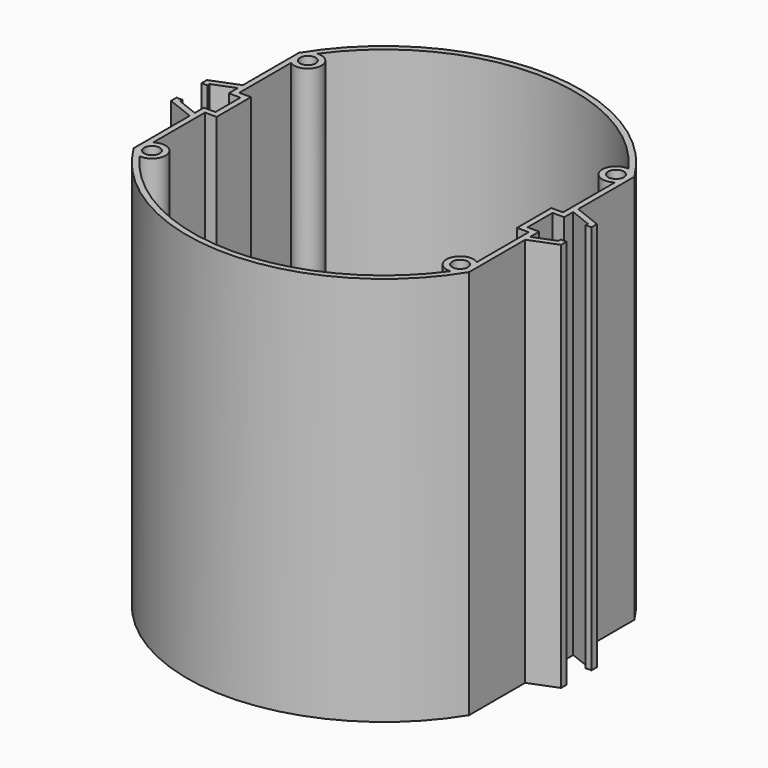
from build123d import *

# Parameters (mm, degrees)
F0_R          = 2
F1_DEPTH      = 100
F1_DEPTH_BACK = 1.5
F2_T          = 1.5
F2_T3_DEPTH   = 104.5
F0_W          = 7
F0_H          = 1.75
F0_H_2        = 8
F0_W_2        = 3
F3_DEPTH      = 100
F3_DEPTH_BACK = 1.5
F4_T          = 1.5
F4_T3_DEPTH   = 104.5
F4_T5_DEPTH   = 103
F4_T7_DEPTH   = 19.6088440305
F4_T9_DEPTH   = 6
F4_T11_DEPTH  = 14
F4_T13_DEPTH  = 19.6088440305
F4_T15_DEPTH  = 6
F4_T18_ANGLE  = 221.2149297422
F4_T20_ANGLE  = 108.9853327241
F4_T22_ANGLE  = 221.2149297422
F4_T24_ANGLE  = 221.2149297422
F4_T26_ANGLE  = 108.9853327241
F4_T28_ANGLE  = 221.2149297422
F0_W_3        = 2
F5_DEPTH      = 1.5
F6_DEPTH      = 100
F6_DEPTH_BACK = 1.5


# Not quite as in the source:
# - a shell that OpenCascade refuses in one call is made with other operations: the cavity is built on its own and cut out


with BuildPart() as f1:
    # F0 (on Top) → F1 (new body, two sides)
    with BuildSketch(Plane.XY) as f1_sk:
        with BuildLine():
            Line((43, 8.5), (43, 26.4811253537))
            ThreePointArc((43, 26.4811253537), (0, 50.5), (-43, 26.4811253537))
            Line((-43, 26.4811253537), (-43, 8.5))
            Line((-43, 8.5), (-43, 5.75))
            Line((-43, 5.75), (-43, 4))
            Line((-43, 4), (-40, 4))
            Line((-40, 4), (-40, -4))
            Line((-40, -4), (-43, -4))
            Line((-43, -4), (-43, -5.75))
            Line((-43, -5.75), (-43, -8.5))
            Line((-43, -8.5), (-43, -26.4811253537))
            ThreePointArc((-43, -26.4811253537), (0, -50.5), (43, -26.4811253537))
            Line((43, -26.4811253537), (43, -8.5))
            Line((43, -8.5), (43, -5.75))
            Line((43, -5.75), (43, -4))
            Line((43, -4), (40, -4))
            Line((40, -4), (40, 4))
            Line((40, 4), (43, 4))
            Line((43, 4), (43, 5.75))
            Line((43, 5.75), (43, 8.5))
        make_face()
        with Locations((-39.5, -24.9811253537)):
            Circle(F0_R, mode=Mode.SUBTRACT)
        with Locations((39.5, -24.9811253537)):
            Circle(F0_R, mode=Mode.SUBTRACT)
        with Locations((-39.5, 24.9811253537)):
            Circle(F0_R, mode=Mode.SUBTRACT)
        with Locations((39.5, 24.9811253537)):
            Circle(F0_R, mode=Mode.SUBTRACT)
    extrude(amount=F1_DEPTH)
    extrude(f1_sk.sketch, amount=-F1_DEPTH_BACK)

    # F2: shell of thickness 1.5, made by hand


with BuildPart() as f2_core1:
    # F2_t2: copy of F1
    add(f1.part)

    # the walls: a layer under each face that stays
    f2_faces = [f2_core1.faces().sort_by_distance(p)[0] for p in [
        (43, -15.2405626769, 49.25),
        (0, 0, -1.5),
        (37.5, 24.9811253537, 49.25),
        (-41.5, 24.9811253537, 49.25),
        (37.5, -24.9811253537, 49.25),
        (-41.5, -24.9811253537, 49.25),
        (-43, -15.2405626769, 49.25),
        (-41.5, -4, 49.25),
        (-40, 0, 49.25),
        (-41.5, 4, 49.25),
        (-43, 15.2405626769, 49.25),
        (0, 50.5, 49.25),
        (43, 15.2405626769, 49.25),
        (41.5, 4, 49.25),
        (40, 0, 49.25),
        (41.5, -4, 49.25),
        (0, -50.5, 49.25),
    ]]
    thicken(f2_faces, amount=-F2_T, mode=Mode.SUBTRACT)

    # F2_s4 → F2_t3 (cut)
    with BuildSketch(Plane.XY.offset(-3)):
        Polygon((-40.015, -3.985), (-40, -5.5), (-38.5, -5.5), (-38.5, -4), align=None)
        Polygon((-40.015, 3.985), (-38.5, 4), (-38.5, 5.5), (-40, 5.5), align=None)
        Polygon((40.015, 3.985), (40, 5.5), (38.5, 5.5), (38.5, 4), align=None)
        Polygon((40.015, -3.985), (38.5, -4), (38.5, -5.5), (40, -5.5), align=None)
    extrude(amount=F2_T3_DEPTH, mode=Mode.SUBTRACT)


with BuildPart() as f1_1:
    add(f1.part)

    # what is left inside the walls is the cavity
    f2_cavity = [f2_core1.part.solids().sort_by_distance(p)[0] for p in [
        (0, -48.985, 66.666667),
    ]]
    add(f2_cavity, mode=Mode.SUBTRACT)

    # F0 (on Top) → F3 (join, two sides)
    with BuildSketch(Plane.XY) as f3_sk:
        Polygon((-43, 5.75), (-43, 8.5), (-50, 5.75), align=None)
        with Locations((-46.5, 4.875)):
            Rectangle(F0_W, F0_H)
        with Locations((-46.5, 0)):
            Rectangle(F0_W, F0_H_2)
        with Locations((-46.5, -4.875)):
            Rectangle(F0_W, F0_H)
        Polygon((-43, -8.5), (-43, -5.75), (-50, -5.75), align=None)
        with Locations((-41.5, 0)):
            Rectangle(F0_W_2, F0_H_2)
        Polygon((50, -5.75), (43, -5.75), (43, -8.5), align=None)
        with Locations((46.5, -4.875)):
            Rectangle(F0_W, F0_H)
        with Locations((46.5, 0)):
            Rectangle(F0_W, F0_H_2)
        with Locations((41.5, 0)):
            Rectangle(F0_W_2, F0_H_2)
        Polygon((50, 5.75), (43, 8.5), (43, 5.75), align=None)
        with Locations((46.5, 4.875)):
            Rectangle(F0_W, F0_H)
    extrude(amount=F3_DEPTH)
    extrude(f3_sk.sketch, amount=-F3_DEPTH_BACK)

    # F4: shell of thickness 1.5, made by hand


with BuildPart() as f4_core1:
    # F4_t2: copy of F1
    add(f1_1.part)

    # the walls: a layer under each face that stays
    f4_faces = [f4_core1.faces().sort_by_distance(p)[0] for p in [
        (43, -17.4905626769, 49.25),
        (0, -50.5, 49.25),
        (0, 0, -1.5),
        (46.5, -7.125, 49.25),
        (-43, -17.4905626769, 49.25),
        (43, 17.4905626769, 49.25),
        (0, 50.5, 49.25),
        (-43, 17.4905626769, 49.25),
        (-41.5, -24.9811253537, 49.25),
        (37.5, -24.9811253537, 49.25),
        (-41.5, 24.9811253537, 49.25),
        (37.5, 24.9811253537, 49.25),
        (50, 0, 49.25),
        (41.5, -13.8044220152, 50),
        (40, -5.5, 50),
        (38.5, 0, 50),
        (40, 5.5, 50),
        (41.5, 13.8044220152, 50),
        (36.1075781641, 24.1200364574, 50),
        (0, 49, 50),
        (-36.1075781641, 24.1200364574, 50),
        (-41.5, 13.8044220152, 50),
        (-40, 5.5, 50),
        (-38.5, 0, 50),
        (-40, -5.5, 50),
        (-41.5, -13.8044220152, 50),
        (-36.1075781641, -24.1200364574, 50),
        (0, -49, 50),
        (36.1075781641, -24.1200364574, 50),
        (-46.5, -7.125, 49.25),
        (46.5, 7.125, 49.25),
        (-46.5, 7.125, 49.25),
        (-50, 0, 49.25),
        (0, 0, 0),
    ]]
    thicken(f4_faces, amount=-F4_T, mode=Mode.SUBTRACT)

    # F4_s4 → F4_t3 (cut)
    with BuildSketch(Plane.XY.offset(-3)):
        Polygon((43.0204847856, -8.5139612724), (41.5, -8.5), (41.5, -7.4776847547), (42.4515214414, -7.1038727598), align=None)
        Polygon((-43.0204847856, -8.5139612724), (-41.5, -8.5), (-41.5, -7.4776847547), (-42.4515214414, -7.1038727598), align=None)
        Polygon((43.0204847856, 8.5139612724), (41.5, 8.5), (41.5, 7.4776847547), (42.4515214414, 7.1038727598), align=None)
        Polygon((-43.0204847856, 8.5139612724), (-41.5, 8.5), (-41.5, 7.4776847547), (-42.4515214414, 7.1038727598), align=None)
    extrude(amount=F4_T3_DEPTH, mode=Mode.SUBTRACT)

    # F4_s6 → F4_t5 (cut)
    with BuildSketch(Plane.XY.offset(-1.5)):
        Polygon((41.4935714286, -22.0965342534), (43, -22.1088440305), (43, -24.9811253537), (40.6428571429, -23.3398217404), align=None)
        Polygon((41.485, -5.515), (43, -5.5), (43, -4), (41.5, -4), align=None)
        Polygon((41.485, 5.515), (41.5, 4), (43, 4), (43, 5.5), align=None)
        Polygon((41.4935714286, 22.0965342534), (43, 22.1088440305), (43, 24.9811253537), (40.6428571429, 23.3398217404), align=None)
        Polygon((39.8774703303, 28.4657460045), (39.7217245792, 26.9687969088), (43.0599998648, 26.5964126076), (41.1090797896, 29.330761307), align=None)
        Polygon((-39.8774703303, 28.4657460045), (-41.1090797896, 29.330761307), (-43.0599998648, 26.5964126076), (-39.7217245792, 26.9687969088), align=None)
        Polygon((-41.4935714286, 22.0965342534), (-40.6428571429, 23.3398217404), (-43, 24.9811253537), (-43, 22.1088440305), align=None)
        Polygon((-41.485, 5.515), (-43, 5.5), (-43, 4), (-41.5, 4), align=None)
        Polygon((-41.485, -5.515), (-41.5, -4), (-43, -4), (-43, -5.5), align=None)
        Polygon((-41.4935714286, -22.0965342534), (-43, -22.1088440305), (-43, -24.9811253537), (-40.6428571429, -23.3398217404), align=None)
        Polygon((-39.8774703303, -28.4657460045), (-39.7217245792, -26.9687969088), (-43.0599998648, -26.5964126076), (-41.1090797896, -29.330761307), align=None)
        Polygon((39.8774703303, -28.4657460045), (41.1090797896, -29.330761307), (43.0599998648, -26.5964126076), (39.7217245792, -26.9687969088), align=None)
    extrude(amount=F4_T5_DEPTH, mode=Mode.SUBTRACT)

    # F4_s8 → F4_t7 (cut)
    with BuildSketch(Plane.XZ.offset(4)):
        Polygon((41.485, 0.015), (43, 0), (43, -1.5), (41.5, -1.5), align=None)
        Polygon((-41.485, 0.015), (-43, 0), (-43, -1.5), (-41.5, -1.5), align=None)
    extrude(amount=F4_T7_DEPTH, mode=Mode.SUBTRACT)

    # F4_s10 → F4_t9 (cut)
    with BuildSketch(Plane.YZ.offset(37)):
        Polygon((-5.515, 0.015), (-4, 0), (-4, -1.5), (-5.5, -1.5), align=None)
        Polygon((5.515, 0.015), (4, 0), (4, -1.5), (5.5, -1.5), align=None)
    extrude(amount=F4_T9_DEPTH, mode=Mode.SUBTRACT)

    # F4_s12 → F4_t11 (cut)
    with BuildSketch(Plane.XZ.offset(-7)):
        Polygon((38.485, 0.015), (40, 0), (40, -1.5), (38.5, -1.5), align=None)
        Polygon((-38.485, 0.015), (-40, 0), (-40, -1.5), (-38.5, -1.5), align=None)
    extrude(amount=F4_T11_DEPTH, mode=Mode.SUBTRACT)

    # F4_s14 → F4_t13 (cut)
    with BuildSketch(Plane.XZ.offset(-23.6088440305)):
        Polygon((41.485, 0.015), (43, 0), (43, -1.5), (41.5, -1.5), align=None)
        Polygon((-41.485, 0.015), (-43, 0), (-43, -1.5), (-41.5, -1.5), align=None)
    extrude(amount=F4_T13_DEPTH, mode=Mode.SUBTRACT)

    # F4_s16 → F4_t15 (cut)
    with BuildSketch(Plane.YZ.offset(-43)):
        Polygon((5.515, 0.015), (4, 0), (4, -1.5), (5.5, -1.5), align=None)
        Polygon((-5.515, 0.015), (-4, 0), (-4, -1.5), (-5.5, -1.5), align=None)
    extrude(amount=F4_T15_DEPTH, mode=Mode.SUBTRACT)

    # F4_s17 → F4_t18 (revolve, cut)
    with BuildSketch(Plane(origin=(38.3167869041, 26.6803857921, 0), x_dir=(0, 0, 1), z_dir=(0.8206518066, 0.5714285714, 0))):
        Polygon((0.015, 5.5856229178), (0, 4.0706229178), (-1.5, 4.0706229178), (-1.5, 5.5706229178), align=None)
    revolve(axis=Axis((39.5, 24.9811253537, 0), (0, 0, -1)), revolution_arc=F4_T18_ANGLE, mode=Mode.SUBTRACT)

    # F4_s19 → F4_t20 (revolve, cut)
    with BuildSketch(Plane(origin=(0, 0, 0), x_dir=(0, 0, 1), z_dir=(-0.5808071546, -0.814041184, 0))):
        Polygon((0.015, 48.985), (0, 50.5), (-1.5, 50.5), (-1.5, 49), align=None)
    revolve(axis=Axis((0, 0, 0), (0, 0, -1)), revolution_arc=F4_T20_ANGLE, mode=Mode.SUBTRACT)

    # F4_s21 → F4_t22 (revolve, cut)
    with BuildSketch(Plane(origin=(-38.3167869041, 26.6803857921, 0), x_dir=(0, 0, 1), z_dir=(-0.8206518066, 0.5714285714, 0))):
        Polygon((0.015, -5.5856229178), (0, -4.0706229178), (-1.5, -4.0706229178), (-1.5, -5.5706229178), align=None)
    revolve(axis=Axis((-39.5, 24.9811253537, 0), (0, 0, 1)), revolution_arc=F4_T22_ANGLE, mode=Mode.SUBTRACT)

    # F4_s23 → F4_t24 (revolve, cut)
    with BuildSketch(Plane(origin=(-36.2621341759, 4.0450377338, 0), x_dir=(0, 0, 1), z_dir=(-0.9938357776, 0.1108622896, 0))):
        Polygon((0.015, -32.7211965802), (0, -31.2061965802), (-1.5, -31.2061965802), (-1.5, -32.7061965802), align=None)
    revolve(axis=Axis((-39.5, -24.9811253537, 0), (0, 0, 1)), revolution_arc=F4_T24_ANGLE, mode=Mode.SUBTRACT)

    # F4_s25 → F4_t26 (revolve, cut)
    with BuildSketch(Plane(origin=(0, 0, 0), x_dir=(0, 0, 1), z_dir=(0.5808071546, 0.814041184, 0))):
        Polygon((0.015, 48.985), (0, 50.5), (-1.5, 50.5), (-1.5, 49), align=None)
    revolve(axis=Axis((0, 0, 0), (0, 0, -1)), revolution_arc=F4_T26_ANGLE, mode=Mode.SUBTRACT)

    # F4_s27 → F4_t28 (revolve, cut)
    with BuildSketch(Plane(origin=(36.2621341759, 4.0450377338, 0), x_dir=(0, 0, 1), z_dir=(0.9938357776, 0.1108622896, 0))):
        Polygon((0.015, 32.7211965802), (0, 31.2061965802), (-1.5, 31.2061965802), (-1.5, 32.7061965802), align=None)
    revolve(axis=Axis((39.5, -24.9811253537, 0), (0, 0, -1)), revolution_arc=F4_T28_ANGLE, mode=Mode.SUBTRACT)


with BuildPart() as f1_2:
    add(f1_1.part)

    # what is left inside the walls is the cavity
    f4_cavity = [f4_core1.part.solids().sort_by_distance(p)[0] for p in [
        (48.485, 0, 66.666667),
        (-48.485, 0, 66.666667),
    ]]
    add(f4_cavity, mode=Mode.SUBTRACT)

    # F0 (on Top) → F5 (cut)
    with BuildSketch(Plane.XY):
        with Locations((-51, 0)):
            Rectangle(F0_W_3, F0_H_2)
        with Locations((-46.5, 0)):
            Rectangle(F0_W, F0_H_2)
        with Locations((-46.5, 4.875)):
            Rectangle(F0_W, F0_H)
        Polygon((-43, 5.75), (-43, 8.5), (-50, 5.75), align=None)
        with Locations((-41.5, 0)):
            Rectangle(F0_W_2, F0_H_2)
        Polygon((-43, -8.5), (-43, -5.75), (-50, -5.75), align=None)
        with BuildLine():
            Line((43, 8.5), (43, 26.4811253537))
            ThreePointArc((43, 26.4811253537), (0, 50.5), (-43, 26.4811253537))
            Line((-43, 26.4811253537), (-43, 8.5))
            Line((-43, 8.5), (-43, 5.75))
            Line((-43, 5.75), (-43, 4))
            Line((-43, 4), (-40, 4))
            Line((-40, 4), (-40, -4))
            Line((-40, -4), (-43, -4))
            Line((-43, -4), (-43, -5.75))
            Line((-43, -5.75), (-43, -8.5))
            Line((-43, -8.5), (-43, -26.4811253537))
            ThreePointArc((-43, -26.4811253537), (0, -50.5), (43, -26.4811253537))
            Line((43, -26.4811253537), (43, -8.5))
            Line((43, -8.5), (43, -5.75))
            Line((43, -5.75), (43, -4))
            Line((43, -4), (40, -4))
            Line((40, -4), (40, 4))
            Line((40, 4), (43, 4))
            Line((43, 4), (43, 5.75))
            Line((43, 5.75), (43, 8.5))
        make_face()
        with Locations((-39.5, -24.9811253537)):
            Circle(F0_R, mode=Mode.SUBTRACT)
        with Locations((39.5, -24.9811253537)):
            Circle(F0_R, mode=Mode.SUBTRACT)
        with Locations((-39.5, 24.9811253537)):
            Circle(F0_R, mode=Mode.SUBTRACT)
        with Locations((39.5, 24.9811253537)):
            Circle(F0_R, mode=Mode.SUBTRACT)
        with Locations((41.5, 0)):
            Rectangle(F0_W_2, F0_H_2)
        with Locations((46.5, 0)):
            Rectangle(F0_W, F0_H_2)
        with Locations((46.5, 4.875)):
            Rectangle(F0_W, F0_H)
        Polygon((50, 5.75), (43, 8.5), (43, 5.75), align=None)
        Polygon((50, -5.75), (43, -5.75), (43, -8.5), align=None)
        with Locations((46.5, -4.875)):
            Rectangle(F0_W, F0_H)
        with Locations((51, 0)):
            Rectangle(F0_W_3, F0_H_2)
        with Locations((-46.5, -4.875)):
            Rectangle(F0_W, F0_H)
        with Locations((-39.5, 24.9811253537)):
            Circle(F0_R)
        with Locations((39.5, 24.9811253537)):
            Circle(F0_R)
        with Locations((39.5, -24.9811253537)):
            Circle(F0_R)
        with Locations((-39.5, -24.9811253537)):
            Circle(F0_R)
    extrude(amount=-F5_DEPTH, mode=Mode.SUBTRACT)

    # F0 (on Top) → F6 (cut, two sides)
    with BuildSketch(Plane.XY) as f6_sk:
        with Locations((-46.5, 0)):
            Rectangle(F0_W, F0_H_2)
        with Locations((46.5, 0)):
            Rectangle(F0_W, F0_H_2)
    extrude(amount=F6_DEPTH, mode=Mode.SUBTRACT)
    extrude(f6_sk.sketch, amount=-F6_DEPTH_BACK, mode=Mode.SUBTRACT)


solid = f1_2.part
